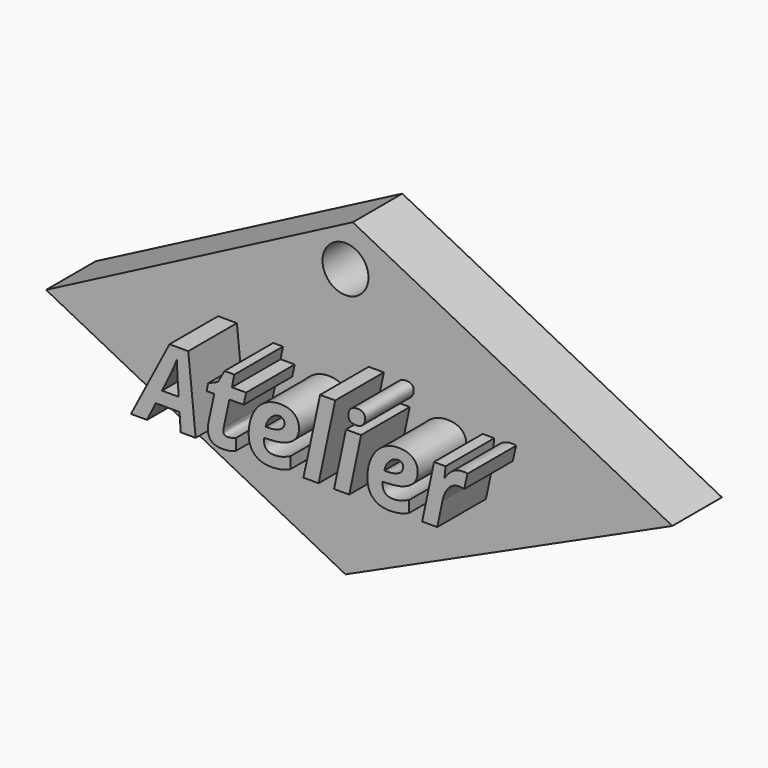
from build123d import *

# Parameters (mm, degrees)
F0_R         = 1.8535791518
F1_DEPTH     = 5
F2_TEXT_SIZE = 8.31890265
F3_DEPTH     = 9.906


# Not quite as in the source:
# - Text() gives the source's letters only with a copy of the font that has no kerning and outlines rounded to 1/6400 em; it was checked with that copy


with BuildPart() as f1:
    # F0 (on Front) → F1 (new body)
    with BuildSketch(Plane.XZ):
        Polygon((36.0484607518, 18.6103843153), (10.2576911449, 31.7988470197), (-14.4876712045, 18.9483734153), (9.6715390682, 6.5942308865), align=None)
        with Locations((9.6715390682, 28.2819233835)):
            Circle(F0_R, mode=Mode.SUBTRACT)
    extrude(amount=F1_DEPTH)

    # F2 (on Front) → F3 (join)
    with BuildSketch(Plane.XZ):
        with Locations((-3.2160193787, 15.6303678889)):
            Text('Atelier', F2_TEXT_SIZE, font='Open Sans', font_style=FontStyle.BOLDITALIC, text_align=(TextAlign.LEFT, TextAlign.BOTTOM))
    extrude(amount=F3_DEPTH)


solid = f1.part
